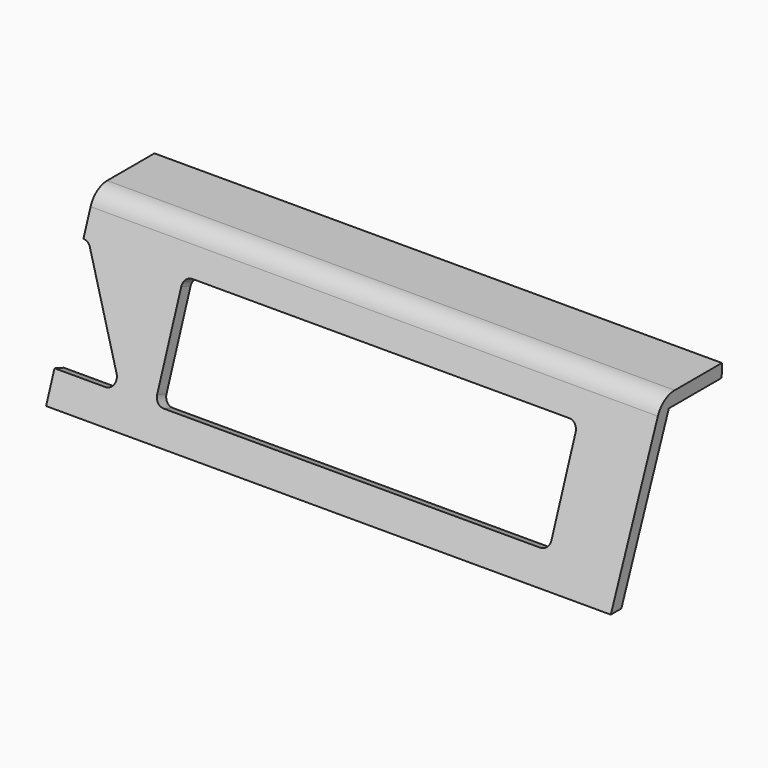
from build123d import *

# Parameters (mm, degrees)
F1_DEPTH = 129
F3_DEPTH = 25
F5_DEPTH = 40
F8_DEPTH = 4


# Not quite as in the source:
# - a feature names something its author has since deleted; it is built from what else it names


with BuildPart() as f1:
    # F0 (on Right) → F1 (new body)
    with BuildSketch(Plane.YZ):
        with BuildLine():
            Line((12.6334434892, 34.7101007166), (0, 0))
            Line((0, 0), (3, 0))
            Line((3, 0), (15.7389581993, 35))
            Line((15.7389581993, 35), (30.7389581993, 35))
            Line((30.7389581993, 35), (30.7389581993, 38))
            Line((30.7389581993, 38), (17.3319065932, 38))
            ThreePointArc((17.3319065932, 38), (14.4640244114, 37.0957602214), (12.6334434892, 34.7101007166))
        make_face()
    extrude(amount=F1_DEPTH)

    # F2 (on face) → F3 (cut)
    with BuildSketch(Plane(origin=(0, 0, 0), x_dir=(1, 0, 0), z_dir=(0, -0.9396926208, 0.3420201433))):
        with BuildLine():
            Line((24.75, 7), (110.25, 7))
            ThreePointArc((110.25, 7), (111.6642135624, 7.5857864376), (112.25, 9))
            Line((112.25, 9), (112.25, 29))
            ThreePointArc((112.25, 29), (111.6642135624, 30.4142135624), (110.25, 31))
            Line((110.25, 31), (24.75, 31))
            ThreePointArc((24.75, 31), (23.3357864376, 30.4142135624), (22.75, 29))
            Line((22.75, 29), (22.75, 9))
            ThreePointArc((22.75, 9), (23.3357864376, 7.5857864376), (24.75, 7))
        make_face()
        with BuildLine():
            ThreePointArc((-13.2679491924, 10), (-13.2679491924, 8), (-11.5358983849, 7))
            Line((-11.5358983849, 7), (0, 7))
            Line((0, 7), (0, 30.9807621135))
            ThreePointArc((0, 30.9807621135), (-1, 30.7128129211), (-1.7320508076, 29.9807621135))
            Line((-1.7320508076, 29.9807621135), (-13.2679491924, 10))
        make_face()
        with BuildLine():
            Line((0, 30.9807621135), (0, 7))
            Line((0, 7), (11.5358983849, 7))
            ThreePointArc((11.5358983849, 7), (13.2679491924, 8), (13.2679491924, 10))
            Line((13.2679491924, 10), (1.7320508076, 29.9807621135))
            ThreePointArc((1.7320508076, 29.9807621135), (1, 30.7128129211), (0, 30.9807621135))
        make_face()
    extrude(amount=-F3_DEPTH, mode=Mode.SUBTRACT)

    # F4 (on Front) → F5 (cut)
    with BuildSketch(Plane.XZ):
        Polygon((149, 50), (129, 50), (128, -10), (149, -10), align=None)
    extrude(amount=-F5_DEPTH, mode=Mode.SUBTRACT)

    # F7 (on offset) → F8 (join)
    with BuildSketch(Plane.YZ.offset(89)):
        Polygon((22.8702962437, 29.2118719039), (13.4733700358, 32.6320733372), (13.1313498925, 31.6923807164), (21.5885834796, 28.6141994265), (22.186255957, 27.3324866624), align=None)
    extrude(amount=F8_DEPTH)


solid = f1.part
